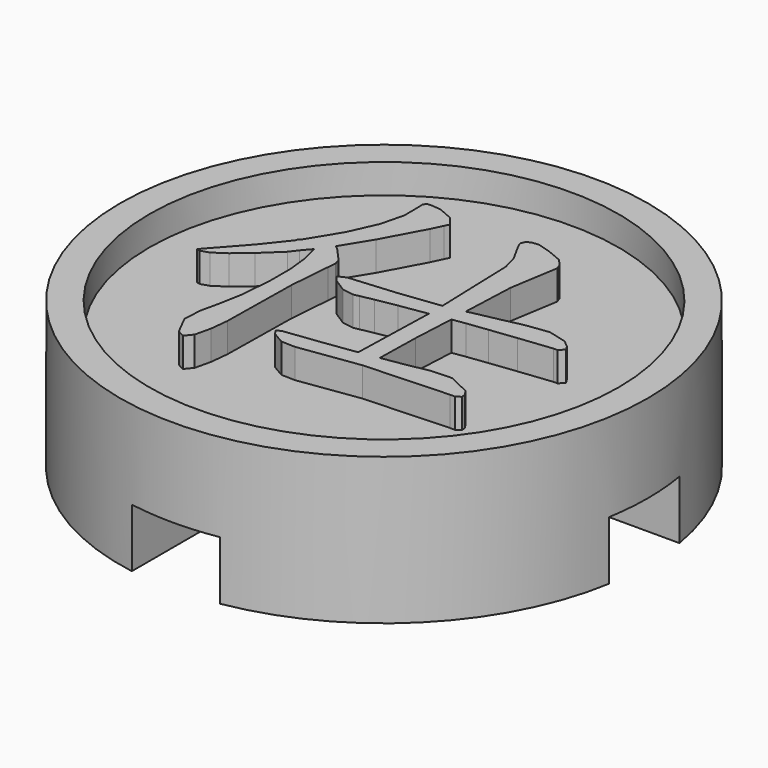
from build123d import *

# Parameters (mm, degrees)
F0_R     = 9
F1_DEPTH = 4
F3_W     = 3
F3_H     = 3
F4_DEPTH = 2
F2_R     = 9
F2_R_2   = 8
F5_DEPTH = 1
F7_DEPTH = 1


# Not quite as in the source:
# - a feature names something its author has since deleted; it is built from what else it names


with BuildPart() as f1:
    # F0 (on Top) → F1 (new body)
    with BuildSketch(Plane.XY):
        with Locations((-31.3306450844, 19.7580661625)):
            Circle(F0_R)
    extrude(amount=F1_DEPTH)

    # F3 (on face) → F4 (cut)
    with BuildSketch(Plane(origin=(0, 0, 0), x_dir=(1, 0, 0), z_dir=(0, 0, -1))):
        with BuildLine():
            ThreePointArc((-32.8306450844, -28.6321858371), (-32.0832814269, -28.7265408676), (-31.3306450844, -28.7580661625))
            ThreePointArc((-31.3306450844, -28.7580661625), (-30.5780087419, -28.7265408676), (-29.8306450844, -28.6321858371))
            Line((-29.8306450844, -28.6321858371), (-29.8306450844, -21.2580661625))
            Line((-29.8306450844, -21.2580661625), (-32.8306450844, -21.2580661625))
            Line((-32.8306450844, -21.2580661625), (-32.8306450844, -28.6321858371))
        make_face()
        with BuildLine():
            ThreePointArc((-40.204764759, -18.2580661625), (-40.2991197895, -19.0054298199), (-40.3306450844, -19.7580661625))
            ThreePointArc((-40.3306450844, -19.7580661625), (-40.2991197895, -20.510702505), (-40.204764759, -21.2580661625))
            Line((-40.204764759, -21.2580661625), (-32.8306450844, -21.2580661625))
            Line((-32.8306450844, -21.2580661625), (-32.8306450844, -18.2580661625))
            Line((-32.8306450844, -18.2580661625), (-40.204764759, -18.2580661625))
        make_face()
        with Locations((-31.3306450844, -19.7580661625)):
            Rectangle(F3_W, F3_H)
        with BuildLine():
            Line((-29.8306450844, -18.2580661625), (-29.8306450844, -21.2580661625))
            Line((-29.8306450844, -21.2580661625), (-22.4565254097, -21.2580661625))
            ThreePointArc((-22.4565254097, -21.2580661625), (-22.3621703793, -20.510702505), (-22.3306450844, -19.7580661625))
            ThreePointArc((-22.3306450844, -19.7580661625), (-22.3621703793, -19.0054298199), (-22.4565254097, -18.2580661625))
            Line((-22.4565254097, -18.2580661625), (-29.8306450844, -18.2580661625))
        make_face()
        with BuildLine():
            Line((-32.8306450844, -10.8839464878), (-32.8306450844, -18.2580661625))
            Line((-32.8306450844, -18.2580661625), (-29.8306450844, -18.2580661625))
            Line((-29.8306450844, -18.2580661625), (-29.8306450844, -10.8839464878))
            ThreePointArc((-29.8306450844, -10.8839464878), (-30.5780087419, -10.7895914574), (-31.3306450844, -10.7580661625))
            ThreePointArc((-31.3306450844, -10.7580661625), (-32.0832814269, -10.7895914574), (-32.8306450844, -10.8839464878))
        make_face()
    extrude(amount=-F4_DEPTH, mode=Mode.SUBTRACT)

    # F2 (on face) → F5 (join)
    with BuildSketch(Plane.XY.offset(4)):
        with Locations((-31.3306450844, 19.7580661625)):
            Circle(F2_R)
        with Locations((-31.3306450844, 19.7580661625)):
            Circle(F2_R_2, mode=Mode.SUBTRACT)
    extrude(amount=F5_DEPTH)

    # F6 (on face) → F7 (join)
    with BuildSketch(Plane.XY.offset(4)):
        Polygon((-34.9050166448, 20.6202120843), (-34.6433972716, 20.9240779367), (-34.5026717981, 20.3743209936), (-34.4223662395, 19.6491017819), (-34.4207141089, 18.7433737938), (-34.5142607427, 17.652222692), (-34.6425682025, 16.9327949487), (-34.7957417285, 16.2514322926), (-34.8255401553, 15.620582776), (-34.5142607427, 15.0062852041), (-34.4480313361, 14.930120185), (-34.2493371085, 14.8407080829), (-34.0506428809, 15.0857628952), (-33.9247925897, 15.6238930448), (-33.8585631831, 16.2381852097), (-33.8179988731, 18.9329782997), (-33.7062427572, 20.331275484), (-33.6789195223, 20.6260155682), (-33.7426497061, 20.8346225789), (-34.1532852441, 21.2949361796), (-34.2956868792, 21.4108256257), (-33.6996102042, 22.3869043351), (-32.9611258864, 23.7554691778), (-32.7839634252, 24.124705329), (-32.7028348052, 24.2952051983), (-32.9478788035, 24.5899452825), (-33.2119733685, 24.7132843353), (-33.4479276451, 24.8085071305), (-33.7319078538, 24.8383055573), (-33.9115455069, 24.8350012963), (-34.0017938873, 24.7356331554), (-33.9877177353, 24.6164394483), (-33.9810851823, 23.9450136062), (-34.1797794099, 23.1461033657), (-34.6028329616, 22.2081137744), (-35.2692903966, 21.1160855415), (-35.3305513962, 21.0697658095), (-35.3355198033, 21.0266902611), (-36.0085977758, 20.1789490503), (-37.0144827221, 19.0496908072), (-37.0782297275, 18.9685621872), (-36.9648088648, 18.947048444), (-36.6833260766, 19.0364677553), (-36.2677239339, 19.31379138), (-35.7353954658, 19.7600288287), (-35.1037108724, 20.357763642), align=None)
        Polygon((-29.9310764641, 19.9206399459), (-30.0105589614, 17.0097722153), (-31.1588076939, 16.8475089676), (-32.3451815909, 16.7018030715), (-32.5140773917, 16.6256428585), (-32.4081067365, 16.4567530655), (-31.9974772062, 16.2150073205), (-31.5239165226, 16.2017602376), (-29.45586365, 16.4940071067), (-26.5731061692, 16.6256428585), (-26.3976198696, 16.6256428585), (-26.2519319967, 16.7282972372), (-26.2618447798, 16.8756552638), (-26.3943156085, 17.059450278), (-27.1311057416, 17.4096598934), (-27.8447660474, 17.3806665048), (-28.563352706, 17.2415931617), (-29.3581176009, 17.1124326018), (-29.3291602587, 18.5935345676), (-29.2555052764, 20.0365474153), (-28.8018001977, 20.1027828296), (-28.1179983962, 20.1897209413), (-27.2114293234, 20.297343727), (-26.0862984027, 20.4239990563), (-25.9414516145, 20.4223409181), (-25.791618396, 20.5895845884), (-25.8826958455, 20.7419230375), (-26.1127925684, 20.9372949808), (-26.746970377, 21.103709582), (-27.5368089191, 21.0001960954), (-28.2669905301, 20.8387679245), (-28.7885831536, 20.731139131), (-29.1114394953, 20.6657327858), (-29.2422281548, 20.629325837), (-29.1661099961, 22.4531697882), (-28.8978640776, 24.103137516), (-28.9649105379, 24.2819881542), (-29.1661099961, 24.5137670463), (-29.6983964099, 24.7356331554), (-30.1131712858, 24.858191201), (-30.3367195641, 24.8408288112), (-30.4973066504, 24.7687959206), (-30.5701806256, 24.6048444959), (-30.4840896063, 24.4110946444), (-30.1521014886, 23.8050931708), (-30.0237760055, 23.3182854043), (-29.9790783653, 21.9216643815), (-29.9310764641, 20.500165277), (-31.318589742, 20.331275484), (-32.9346317206, 20.1921961332), (-33.203712716, 20.0646937115), (-33.0372981148, 19.8709618832), (-32.5910546583, 19.5845245058), (-32.2027799559, 19.5232514908), (-32.0107242891, 19.5629927394), (-31.5628287021, 19.6507539124), (-30.8673838862, 19.7741049807), align=None)
    extrude(amount=F7_DEPTH)


solid = f1.part
